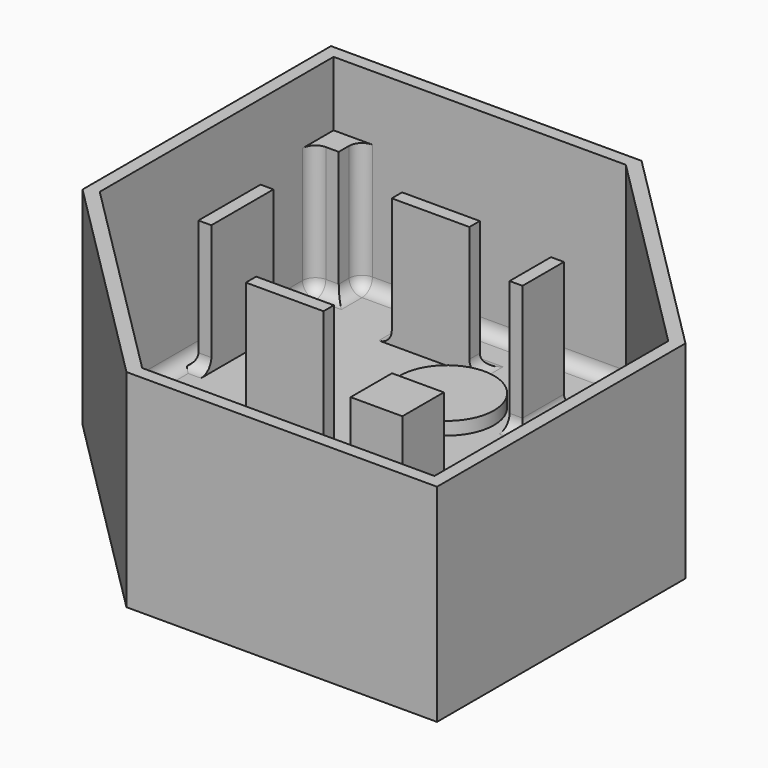
from build123d import *

# Parameters (mm, degrees)
F1_DEPTH      = 50.8
F2_T          = -3.175
F3_W          = 19.05
F3_H          = 3.175
F3_W_2        = 3.175
F3_H_2        = 19.05
F3_H_3        = 12.7
F3_W_3        = 12.7
F3_W_4        = 6.35
F3_H_4        = 6.35
F4_DEPTH      = 31.75
F5_R          = 11.557
F6_DEPTH      = 3.175
F7_T1_DEPTH   = 12.7
F7_T3_DEPTH   = 3.175
F7_T5_DEPTH   = 19.05
F7_T7_DEPTH   = 3.175
F7_T9_DEPTH   = 3.175
F7_T11_DEPTH  = 19.05
F7_T13_DEPTH  = 3.175
F7_T15_DEPTH  = 12.7
F7_T17_DEPTH  = 12.7
F7_T19_DEPTH  = 3.175
F7_T21_DEPTH  = 3.175
F7_T23_DEPTH  = 3.175
F7_T25_DEPTH  = 3.175
F7_T27_DEPTH  = 28.575
F7_S31_W      = 3.2385
F7_S31_H      = 3.2385
F7_T32_DEPTH  = 3.2385
F7_S37_W      = 3.2385
F7_S37_H      = 3.2385
F7_T38_DEPTH  = 3.2385
F7_S43_W      = 3.2385
F7_S43_H      = 3.2385
F7_T44_DEPTH  = 3.2385
F7_S49_W      = 3.2385
F7_S49_H      = 3.2385
F7_T50_DEPTH  = 3.2385
F7_T56_DEPTH  = 70.1223719395
F7_T61_DEPTH  = 89.4447438789
F7_T67_DEPTH  = 70.1223719395
F7_T72_DEPTH  = 70.1223719395
F7_T77_DEPTH  = 89.4447438789
F7_T83_DEPTH  = 70.1223719395
F7_T89_DEPTH  = 11.1125
F7_T93_DEPTH  = 20.6375
F7_T100_DEPTH = 11.1125
F7_T104_DEPTH = 20.6375
F7_T111_DEPTH = 26.9875
F7_T115_DEPTH = 11.1125
F7_T122_DEPTH = 26.9875
F7_T126_DEPTH = 11.1125
F7_T133_DEPTH = 26.9875
F7_T137_DEPTH = 11.1125
F7_T145_DEPTH = 26.9875
F7_T149_DEPTH = 11.1125
F7_T157_DEPTH = 11.1125
F7_T161_DEPTH = 26.9875
F7_T168_DEPTH = 26.9875
F7_T172_DEPTH = 11.1125
F7_T179_DEPTH = 20.6375
F7_T183_DEPTH = 20.6375
F7_T190_DEPTH = 20.6375
F7_T194_DEPTH = 20.6375
F7_T201_DEPTH = 20.6375
F7_T205_DEPTH = 20.6375
F7_T212_DEPTH = 20.6375
F7_T216_DEPTH = 20.6375
F7_T223_DEPTH = 11.1125
F7_T227_DEPTH = 11.1125
F7_T234_DEPTH = 11.1125
F7_T238_DEPTH = 11.1125


# Not quite as in the source:
# - a fillet or chamfer that OpenCascade refuses, or shapes differently, is made with other operations: its cross-section is extruded or revolved along the edge and cut away or added


with BuildPart() as f1:
    # F0 (on Top) → F1 (new body)
    with BuildSketch(Plane.XY):
        Polygon((-53.8815367264, 53.8815367264), (0, 0), (76.2, 0), (76.2, 76.2), (22.3184632736, 130.0815367264), (-53.8815367264, 130.0815367264), align=None)
    extrude(amount=F1_DEPTH)

    # F2
    f2_openings = [f1.faces().sort_by_distance(p)[0] for p in [
        (11.159232, 65.040768, 50.8),
    ]]
    offset(amount=F2_T, openings=f2_openings)

    # F3 (on face) → F4 (join)
    with BuildSketch(Plane.XY.offset(3.175)):
        with Locations((-14.8516007567, 113.4290007567)):
            Rectangle(F3_W, F3_H)
        with Locations((-14.8516007567, 68.6742007567)):
            Rectangle(F3_W, F3_H)
        with Locations((-45.9793007567, 91.0516007567)):
            Rectangle(F3_W_2, F3_H_2)
        with Locations((16.2760992433, 105.4915007567)):
            Rectangle(F3_W_2, F3_H_3)
        with Locations((27.3533352131, 48.8466647869)):
            Rectangle(F3_W_3, F3_H_3)
        with Locations((69.85, 6.35)):
            Rectangle(F3_W_4, F3_H_4)
        with Locations((-47.5315367264, 123.7315367264)):
            Rectangle(F3_W_4, F3_H_4)
    extrude(amount=F4_DEPTH)

    # F5 (on face) → F6 (join)
    with BuildSketch(Plane.XY.offset(3.175)):
        with Locations((0.0581992433, 98.2017007567)):
            Circle(F5_R)
    extrude(amount=F6_DEPTH)

    # F7: fillet of radius 3.175 on 30 edges, made by hand

    # F7_s2 → F7_t1 (join)
    with BuildSketch(Plane.XZ.offset(-111.8415007567)):
        with BuildLine():
            ThreePointArc((21.0385992433, 3.175), (18.7935352131, 4.1049359697), (17.8635992433, 6.35))
            Line((17.8635992433, 6.35), (17.8635992433, 3.175))
            Line((17.8635992433, 3.175), (21.0385992433, 3.175))
        make_face()
    extrude(amount=F7_T1_DEPTH)

    # F7_s4 → F7_t3 (join)
    with BuildSketch(Plane.YZ.offset(14.6885992433)):
        with BuildLine():
            ThreePointArc((115.0165007567, 3.175), (112.7714367264, 4.1049359697), (111.8415007567, 6.35))
            Line((111.8415007567, 6.35), (111.8415007567, 3.175))
            Line((111.8415007567, 3.175), (115.0165007567, 3.175))
        make_face()
        with BuildLine():
            ThreePointArc((95.9665007567, 3.175), (98.2115647869, 4.1049359697), (99.1415007567, 6.35))
            Line((99.1415007567, 6.35), (99.1415007567, 3.175))
            Line((99.1415007567, 3.175), (95.9665007567, 3.175))
        make_face()
    extrude(amount=F7_T3_DEPTH)

    # F7_s6 → F7_t5 (join)
    with BuildSketch(Plane.YZ.offset(-24.3766007567)):
        with BuildLine():
            ThreePointArc((63.9117007567, 3.175), (66.1567647869, 4.1049359697), (67.0867007567, 6.35))
            Line((67.0867007567, 6.35), (67.0867007567, 3.175))
            Line((67.0867007567, 3.175), (63.9117007567, 3.175))
        make_face()
        with BuildLine():
            ThreePointArc((118.1915007567, 3.175), (115.9464367264, 4.1049359697), (115.0165007567, 6.35))
            Line((115.0165007567, 6.35), (115.0165007567, 3.175))
            Line((115.0165007567, 3.175), (118.1915007567, 3.175))
        make_face()
    extrude(amount=F7_T5_DEPTH)

    # F7_s8 → F7_t7 (join)
    with BuildSketch(Plane.XZ.offset(-70.2617007567)):
        with BuildLine():
            ThreePointArc((-2.1516007567, 3.175), (-4.3966647869, 4.1049359697), (-5.3266007567, 6.35))
            Line((-5.3266007567, 6.35), (-5.3266007567, 3.175))
            Line((-5.3266007567, 3.175), (-2.1516007567, 3.175))
        make_face()
        with BuildLine():
            ThreePointArc((-27.5516007567, 3.175), (-25.3065367264, 4.1049359697), (-24.3766007567, 6.35))
            Line((-24.3766007567, 6.35), (-24.3766007567, 3.175))
            Line((-24.3766007567, 3.175), (-27.5516007567, 3.175))
        make_face()
    extrude(amount=F7_T7_DEPTH)

    # F7_s10 → F7_t9 (join)
    with BuildSketch(Plane.YZ.offset(-47.5668007567)):
        with BuildLine():
            ThreePointArc((78.3516007567, 3.175), (80.5966647869, 4.1049359697), (81.5266007567, 6.35))
            Line((81.5266007567, 6.35), (81.5266007567, 3.175))
            Line((81.5266007567, 3.175), (78.3516007567, 3.175))
        make_face()
        with BuildLine():
            ThreePointArc((103.7516007567, 3.175), (101.5065367264, 4.1049359697), (100.5766007567, 6.35))
            Line((100.5766007567, 6.35), (100.5766007567, 3.175))
            Line((100.5766007567, 3.175), (103.7516007567, 3.175))
        make_face()
    extrude(amount=F7_T9_DEPTH)

    # F7_s12 → F7_t11 (join)
    with BuildSketch(Plane.XZ.offset(-100.5766007567)):
        with BuildLine():
            ThreePointArc((-50.7418007567, 3.175), (-48.4967367264, 4.1049359697), (-47.5668007567, 6.35))
            Line((-47.5668007567, 6.35), (-47.5668007567, 3.175))
            Line((-47.5668007567, 3.175), (-50.7418007567, 3.175))
        make_face()
    extrude(amount=F7_T11_DEPTH)

    # F7_s14 → F7_t13 (join)
    with BuildSketch(Plane.XZ.offset(-115.0165007567)):
        with BuildLine():
            ThreePointArc((-27.5516007567, 3.175), (-25.3065367264, 4.1049359697), (-24.3766007567, 6.35))
            Line((-24.3766007567, 6.35), (-24.3766007567, 3.175))
            Line((-24.3766007567, 3.175), (-27.5516007567, 3.175))
        make_face()
        with BuildLine():
            ThreePointArc((-2.1516007567, 3.175), (-4.3966647869, 4.1049359697), (-5.3266007567, 6.35))
            Line((-5.3266007567, 6.35), (-5.3266007567, 3.175))
            Line((-5.3266007567, 3.175), (-2.1516007567, 3.175))
        make_face()
    extrude(amount=F7_T13_DEPTH)

    # F7_s16 → F7_t15 (join)
    with BuildSketch(Plane.YZ.offset(21.0033352131)):
        with BuildLine():
            ThreePointArc((58.3716647869, 3.175), (56.1266007567, 4.1049359697), (55.1966647869, 6.35))
            Line((55.1966647869, 6.35), (55.1966647869, 3.175))
            Line((55.1966647869, 3.175), (58.3716647869, 3.175))
        make_face()
        with BuildLine():
            ThreePointArc((39.3216647869, 3.175), (41.5667288172, 4.1049359697), (42.4966647869, 6.35))
            Line((42.4966647869, 6.35), (42.4966647869, 3.175))
            Line((42.4966647869, 3.175), (39.3216647869, 3.175))
        make_face()
    extrude(amount=F7_T15_DEPTH)

    # F7_s18 → F7_t17 (join)
    with BuildSketch(Plane.XZ.offset(-55.1966647869)):
        with BuildLine():
            ThreePointArc((36.8783352131, 3.175), (34.6332711828, 4.1049359697), (33.7033352131, 6.35))
            Line((33.7033352131, 6.35), (33.7033352131, 3.175))
            Line((33.7033352131, 3.175), (36.8783352131, 3.175))
        make_face()
        with BuildLine():
            ThreePointArc((17.8283352131, 3.175), (20.0733992433, 4.1049359697), (21.0033352131, 6.35))
            Line((21.0033352131, 6.35), (21.0033352131, 3.175))
            Line((21.0033352131, 3.175), (17.8283352131, 3.175))
        make_face()
    extrude(amount=F7_T17_DEPTH)

    # F7_s20 → F7_t19 (join)
    with BuildSketch(Plane.YZ.offset(-47.5315367264)):
        with BuildLine():
            ThreePointArc((117.3815367264, 3.175), (119.6266007567, 4.1049359697), (120.5565367264, 6.35))
            Line((120.5565367264, 6.35), (120.5565367264, 3.175))
            Line((120.5565367264, 3.175), (117.3815367264, 3.175))
        make_face()
    extrude(amount=F7_T19_DEPTH)

    # F7_s22 → F7_t21 (join)
    with BuildSketch(Plane.XZ.offset(-123.7315367264)):
        with BuildLine():
            ThreePointArc((-41.1815367264, 3.175), (-43.4266007567, 4.1049359697), (-44.3565367264, 6.35))
            Line((-44.3565367264, 6.35), (-44.3565367264, 3.175))
            Line((-44.3565367264, 3.175), (-41.1815367264, 3.175))
        make_face()
    extrude(amount=F7_T21_DEPTH)

    # F7_s24 → F7_t23 (join)
    with BuildSketch(Plane.YZ.offset(66.675)):
        with BuildLine():
            ThreePointArc((12.7, 3.175), (10.4549359697, 4.1049359697), (9.525, 6.35))
            Line((9.525, 6.35), (9.525, 3.175))
            Line((9.525, 3.175), (12.7, 3.175))
        make_face()
    extrude(amount=F7_T23_DEPTH)

    # F7_s26 → F7_t25 (join)
    with BuildSketch(Plane.XZ.offset(-9.525)):
        with BuildLine():
            ThreePointArc((63.5, 3.175), (65.7450640303, 4.1049359697), (66.675, 6.35))
            Line((66.675, 6.35), (66.675, 3.175))
            Line((66.675, 3.175), (63.5, 3.175))
        make_face()
    extrude(amount=F7_T25_DEPTH)

    # F7_s28 → F7_t27 (join)
    with BuildSketch(Plane.XY.offset(6.35)):
        with BuildLine():
            ThreePointArc((-50.7065367264, 117.3815367264), (-49.7766007567, 119.6266007567), (-47.5315367264, 120.5565367264))
            Line((-47.5315367264, 120.5565367264), (-50.7065367264, 120.5565367264))
            Line((-50.7065367264, 120.5565367264), (-50.7065367264, 117.3815367264))
        make_face()
        with BuildLine():
            ThreePointArc((-41.1815367264, 126.9065367264), (-43.4266007567, 125.9766007567), (-44.3565367264, 123.7315367264))
            Line((-44.3565367264, 123.7315367264), (-44.3565367264, 126.9065367264))
            Line((-44.3565367264, 126.9065367264), (-41.1815367264, 126.9065367264))
        make_face()
        with BuildLine():
            ThreePointArc((73.025, 12.7), (72.0950640303, 10.4549359697), (69.85, 9.525))
            Line((69.85, 9.525), (73.025, 9.525))
            Line((73.025, 9.525), (73.025, 12.7))
        make_face()
        with BuildLine():
            ThreePointArc((63.5, 3.175), (65.7450640303, 4.1049359697), (66.675, 6.35))
            Line((66.675, 6.35), (66.675, 3.175))
            Line((66.675, 3.175), (63.5, 3.175))
        make_face()
    extrude(amount=F7_T27_DEPTH)


with BuildPart() as f7_tool30:
    # F7_s31 → F7_t32 (new body)
    with BuildSketch(Plane.XZ.offset(-117.3815367264)):
        with Locations((-49.1507867264, 4.73075)):
            Rectangle(F7_S31_W, F7_S31_H)
    extrude(amount=-F7_T32_DEPTH)

    # F7_s33 → F7_t34 (revolve, cut)
    with BuildSketch(Plane(origin=(-47.5315367264, 117.3815367264, 6.35), x_dir=(0.7071067812, 0, 0.7071067812), z_dir=(-0.7071067812, 0, 0.7071067812))):
        with BuildLine():
            ThreePointArc((0, -3.175), (3.175, 0), (0, 3.175))
            Line((0, 3.175), (0, -3.175))
        make_face()
    revolve(axis=Axis((-47.5315367264, 117.3815367264, 6.35), (0, 1, 0)), mode=Mode.SUBTRACT)


with BuildPart() as f1_1:
    add(f1.part)

    # F7_t29: union F7_tool30
    add(f7_tool30.part)


with BuildPart() as f7_tool36:
    # F7_s37 → F7_t38 (new body)
    with BuildSketch(Plane.YZ.offset(-41.1815367264)):
        with Locations((125.3507867264, 4.73075)):
            Rectangle(F7_S37_W, F7_S37_H)
    extrude(amount=-F7_T38_DEPTH)

    # F7_s39 → F7_t40 (revolve, cut)
    with BuildSketch(Plane(origin=(-41.1815367264, 123.7315367264, 6.35), x_dir=(0, -0.7071067812, 0.7071067812), z_dir=(0, -0.7071067812, -0.7071067812))):
        with BuildLine():
            ThreePointArc((0, -3.175), (3.175, 0), (0, 3.175))
            Line((0, 3.175), (0, -3.175))
        make_face()
    revolve(axis=Axis((-41.1815367264, 123.7315367264, 6.35), (-1, 0, 0)), mode=Mode.SUBTRACT)


with BuildPart() as f1_2:
    add(f1_1.part)

    # F7_t35: union F7_tool36
    add(f7_tool36.part)


with BuildPart() as f7_tool42:
    # F7_s43 → F7_t44 (new body)
    with BuildSketch(Plane.XZ.offset(-12.7)):
        with Locations((71.46925, 4.73075)):
            Rectangle(F7_S43_W, F7_S43_H)
    extrude(amount=F7_T44_DEPTH)

    # F7_s45 → F7_t46 (revolve, cut)
    with BuildSketch(Plane(origin=(69.85, 12.7, 6.35), x_dir=(-0.7071067812, 0, 0.7071067812), z_dir=(0.7071067812, 0, 0.7071067812))):
        with BuildLine():
            ThreePointArc((0, -3.175), (3.175, 0), (0, 3.175))
            Line((0, 3.175), (0, -3.175))
        make_face()
    revolve(axis=Axis((69.85, 12.7, 6.35), (0, -1, 0)), mode=Mode.SUBTRACT)


with BuildPart() as f1_3:
    add(f1_2.part)

    # F7_t41: union F7_tool42
    add(f7_tool42.part)


with BuildPart() as f7_tool48:
    # F7_s49 → F7_t50 (new body)
    with BuildSketch(Plane.YZ.offset(63.5)):
        with Locations((4.73075, 4.73075)):
            Rectangle(F7_S49_W, F7_S49_H)
    extrude(amount=F7_T50_DEPTH)

    # F7_s51 → F7_t52 (revolve, cut)
    with BuildSketch(Plane(origin=(63.5, 6.35, 6.35), x_dir=(0, 0.7071067812, 0.7071067812), z_dir=(0, 0.7071067812, -0.7071067812))):
        with BuildLine():
            ThreePointArc((0, -3.175), (3.175, 0), (0, 3.175))
            Line((0, 3.175), (0, -3.175))
        make_face()
    revolve(axis=Axis((63.5, 6.35, 6.35), (1, 0, 0)), mode=Mode.SUBTRACT)


with BuildPart() as f1_4:
    add(f1_3.part)

    # F7_t47: union F7_tool48
    add(f7_tool48.part)


with BuildPart() as f7_tool54:
    # F7_s55 → F7_t56 (new body)
    with BuildSketch(Plane.YZ.offset(28.9408352131)):
        with BuildLine():
            ThreePointArc((126.9065367264, 6.35), (125.9766007567, 4.1049359697), (123.7315367264, 3.175))
            Line((123.7315367264, 3.175), (126.9065367264, 3.175))
            Line((126.9065367264, 3.175), (126.9065367264, 6.35))
        make_face()
    extrude(amount=-F7_T56_DEPTH)

    split(bisect_by=Plane(origin=(73.9549359697, 73.9549359697, 0), x_dir=(0, 0, 1), z_dir=(-0.7071067812, -0.7071067812, 0)), keep=Keep.TOP)


with BuildPart() as f1_5:
    add(f1_4.part)

    # F7_t53: union F7_tool54
    add(f7_tool54.part)


with BuildPart() as f7_tool59:
    # F7_s60 → F7_t61 (new body)
    with BuildSketch(Plane(origin=(4.6827241059, -4.6827241059, 0), x_dir=(0, 0, 1), z_dir=(-0.7071067812, 0.7071067812, 0))):
        with BuildLine():
            ThreePointArc((6.35, 104.5880734528), (4.1049359697, 103.6581374831), (3.175, 101.4130734528))
            Line((3.175, 101.4130734528), (3.175, 104.5880734528))
            Line((3.175, 104.5880734528), (6.35, 104.5880734528))
        make_face()
    extrude(amount=F7_T61_DEPTH)

    split(bisect_by=Plane.XZ.offset(-126.9065367264), keep=Keep.TOP)

    split(bisect_by=Plane.YZ.offset(73.025), keep=Keep.BOTTOM)


with BuildPart() as f1_6:
    add(f1_5.part)

    # F7_t58: union F7_tool59
    add(f7_tool59.part)


with BuildPart() as f7_tool65:
    # F7_s66 → F7_t67 (new body)
    with BuildSketch(Plane.XZ.offset(-12.7)):
        with BuildLine():
            ThreePointArc((73.025, 6.35), (72.0950640303, 4.1049359697), (69.85, 3.175))
            Line((69.85, 3.175), (73.025, 3.175))
            Line((73.025, 3.175), (73.025, 6.35))
        make_face()
    extrude(amount=-F7_T67_DEPTH)

    split(bisect_by=Plane(origin=(73.9549359697, 73.9549359697, 0), x_dir=(0, 0, 1), z_dir=(-0.7071067812, -0.7071067812, 0)), keep=Keep.TOP)


with BuildPart() as f1_7:
    add(f1_6.part)

    # F7_t64: union F7_tool65
    add(f7_tool65.part)


with BuildPart() as f7_tool70:
    # F7_s71 → F7_t72 (new body)
    with BuildSketch(Plane.YZ.offset(-6.6223719395)):
        with BuildLine():
            ThreePointArc((3.175, 6.35), (4.1049359697, 4.1049359697), (6.35, 3.175))
            Line((6.35, 3.175), (3.175, 3.175))
            Line((3.175, 3.175), (3.175, 6.35))
        make_face()
    extrude(amount=F7_T72_DEPTH)

    split(bisect_by=Plane(origin=(2.2450640303, 2.2450640303, 0), x_dir=(0, 0, 1), z_dir=(0.7071067812, 0.7071067812, 0)), keep=Keep.TOP)


with BuildPart() as f1_8:
    add(f1_7.part)

    # F7_t69: union F7_tool70
    add(f7_tool70.part)


with BuildPart() as f7_tool75:
    # F7_s76 → F7_t77 (new body)
    with BuildSketch(Plane(origin=(-58.5642608324, 58.5642608324, 0), x_dir=(0, 0, 1), z_dir=(0.7071067812, -0.7071067812, 0))):
        with BuildLine():
            ThreePointArc((6.35, -3.175), (4.1049359697, -4.1049359697), (3.175, -6.35))
            Line((3.175, -6.35), (3.175, -3.175))
            Line((3.175, -3.175), (6.35, -3.175))
        make_face()
    extrude(amount=F7_T77_DEPTH)

    split(bisect_by=Plane.YZ.offset(-50.7065367264), keep=Keep.TOP)

    split(bisect_by=Plane.XZ.offset(-3.175), keep=Keep.BOTTOM)


with BuildPart() as f1_9:
    add(f1_8.part)

    # F7_t74: union F7_tool75
    add(f7_tool75.part)


with BuildPart() as f7_tool81:
    # F7_s82 → F7_t83 (new body)
    with BuildSketch(Plane.XZ.offset(-117.3815367264)):
        with BuildLine():
            ThreePointArc((-50.7065367264, 6.35), (-49.7766007567, 4.1049359697), (-47.5315367264, 3.175))
            Line((-47.5315367264, 3.175), (-50.7065367264, 3.175))
            Line((-50.7065367264, 3.175), (-50.7065367264, 6.35))
        make_face()
    extrude(amount=F7_T83_DEPTH)

    split(bisect_by=Plane(origin=(2.2450640303, 2.2450640303, 0), x_dir=(0, 0, 1), z_dir=(0.7071067812, 0.7071067812, 0)), keep=Keep.TOP)


with BuildPart() as f1_10:
    add(f1_9.part)

    # F7_t80: union F7_tool81
    add(f7_tool81.part)


with BuildPart() as f7_tool87:
    # F7_s88 → F7_t89 (new body)
    with BuildSketch(Plane.YZ.offset(14.6885992433)):
        with BuildLine():
            ThreePointArc((95.9665007567, 3.175), (98.2115647869, 4.1049359697), (99.1415007567, 6.35))
            Line((99.1415007567, 6.35), (99.1415007567, 3.175))
            Line((99.1415007567, 3.175), (95.9665007567, 3.175))
        make_face()
    extrude(amount=F7_T89_DEPTH)

    split(bisect_by=Plane.YZ.offset(17.8635992433), keep=Keep.TOP)


with BuildPart() as f7_tool91:
    # F7_s92 → F7_t93 (new body)
    with BuildSketch(Plane.XZ.offset(-91.2040007567)):
        with BuildLine():
            ThreePointArc((21.0385992433, 3.175), (18.7935352131, 4.1049359697), (17.8635992433, 6.35))
            Line((17.8635992433, 6.35), (17.8635992433, 3.175))
            Line((17.8635992433, 3.175), (21.0385992433, 3.175))
        make_face()
    extrude(amount=-F7_T93_DEPTH)

    split(bisect_by=Plane.XZ.offset(-99.1415007567), keep=Keep.TOP)


with BuildPart() as f7_tool87_1:
    add(f7_tool87.part)

    # F7_t95: intersect F7_tool91
    add(f7_tool91.part, mode=Mode.INTERSECT)


with BuildPart() as f1_11:
    add(f1_10.part)

    # F7_t85: union F7_tool87
    add(f7_tool87_1.part)


with BuildPart() as f7_tool98:
    # F7_s99 → F7_t100 (new body)
    with BuildSketch(Plane.YZ.offset(25.8010992433)):
        with BuildLine():
            ThreePointArc((115.0165007567, 3.175), (112.7714367264, 4.1049359697), (111.8415007567, 6.35))
            Line((111.8415007567, 6.35), (111.8415007567, 3.175))
            Line((111.8415007567, 3.175), (115.0165007567, 3.175))
        make_face()
    extrude(amount=-F7_T100_DEPTH)

    split(bisect_by=Plane.YZ.offset(17.8635992433), keep=Keep.TOP)


with BuildPart() as f7_tool102:
    # F7_s103 → F7_t104 (new body)
    with BuildSketch(Plane.XZ.offset(-99.1415007567)):
        with BuildLine():
            ThreePointArc((21.0385992433, 3.175), (18.7935352131, 4.1049359697), (17.8635992433, 6.35))
            Line((17.8635992433, 6.35), (17.8635992433, 3.175))
            Line((17.8635992433, 3.175), (21.0385992433, 3.175))
        make_face()
    extrude(amount=-F7_T104_DEPTH)

    split(bisect_by=Plane.XZ.offset(-111.8415007567), keep=Keep.BOTTOM)


with BuildPart() as f7_tool98_1:
    add(f7_tool98.part)

    # F7_t106: intersect F7_tool102
    add(f7_tool102.part, mode=Mode.INTERSECT)


with BuildPart() as f1_12:
    add(f1_11.part)

    # F7_t96: union F7_tool98
    add(f7_tool98_1.part)


with BuildPart() as f7_tool109:
    # F7_s110 → F7_t111 (new body)
    with BuildSketch(Plane.YZ.offset(-32.3141007567)):
        with BuildLine():
            ThreePointArc((63.9117007567, 3.175), (66.1567647869, 4.1049359697), (67.0867007567, 6.35))
            Line((67.0867007567, 6.35), (67.0867007567, 3.175))
            Line((67.0867007567, 3.175), (63.9117007567, 3.175))
        make_face()
    extrude(amount=F7_T111_DEPTH)

    split(bisect_by=Plane.YZ.offset(-24.3766007567), keep=Keep.BOTTOM)


with BuildPart() as f7_tool113:
    # F7_s114 → F7_t115 (new body)
    with BuildSketch(Plane.XZ.offset(-70.2617007567)):
        with BuildLine():
            ThreePointArc((-27.5516007567, 3.175), (-25.3065367264, 4.1049359697), (-24.3766007567, 6.35))
            Line((-24.3766007567, 6.35), (-24.3766007567, 3.175))
            Line((-24.3766007567, 3.175), (-27.5516007567, 3.175))
        make_face()
    extrude(amount=F7_T115_DEPTH)

    split(bisect_by=Plane.XZ.offset(-67.0867007567), keep=Keep.TOP)


with BuildPart() as f7_tool109_1:
    add(f7_tool109.part)

    # F7_t117: intersect F7_tool113
    add(f7_tool113.part, mode=Mode.INTERSECT)


with BuildPart() as f1_13:
    add(f1_12.part)

    # F7_t107: union F7_tool109
    add(f7_tool109_1.part)


with BuildPart() as f7_tool120:
    # F7_s121 → F7_t122 (new body)
    with BuildSketch(Plane.YZ.offset(-24.3766007567)):
        with BuildLine():
            ThreePointArc((63.9117007567, 3.175), (66.1567647869, 4.1049359697), (67.0867007567, 6.35))
            Line((67.0867007567, 6.35), (67.0867007567, 3.175))
            Line((67.0867007567, 3.175), (63.9117007567, 3.175))
        make_face()
    extrude(amount=F7_T122_DEPTH)

    split(bisect_by=Plane.YZ.offset(-5.3266007567), keep=Keep.TOP)


with BuildPart() as f7_tool124:
    # F7_s125 → F7_t126 (new body)
    with BuildSketch(Plane.XZ.offset(-59.1492007567)):
        with BuildLine():
            ThreePointArc((-2.1516007567, 3.175), (-4.3966647869, 4.1049359697), (-5.3266007567, 6.35))
            Line((-5.3266007567, 6.35), (-5.3266007567, 3.175))
            Line((-5.3266007567, 3.175), (-2.1516007567, 3.175))
        make_face()
    extrude(amount=-F7_T126_DEPTH)

    split(bisect_by=Plane.XZ.offset(-67.0867007567), keep=Keep.TOP)


with BuildPart() as f7_tool120_1:
    add(f7_tool120.part)

    # F7_t128: intersect F7_tool124
    add(f7_tool124.part, mode=Mode.INTERSECT)


with BuildPart() as f1_14:
    add(f1_13.part)

    # F7_t118: union F7_tool120
    add(f7_tool120_1.part)


with BuildPart() as f7_tool131:
    # F7_s132 → F7_t133 (new body)
    with BuildSketch(Plane.XZ.offset(-100.5766007567)):
        with BuildLine():
            ThreePointArc((-50.7418007567, 3.175), (-48.4967367264, 4.1049359697), (-47.5668007567, 6.35))
            Line((-47.5668007567, 6.35), (-47.5668007567, 3.175))
            Line((-47.5668007567, 3.175), (-50.7418007567, 3.175))
        make_face()
    extrude(amount=F7_T133_DEPTH)

    split(bisect_by=Plane.XZ.offset(-81.5266007567), keep=Keep.TOP)


with BuildPart() as f7_tool135:
    # F7_s136 → F7_t137 (new body)
    with BuildSketch(Plane.YZ.offset(-55.5043007567)):
        with BuildLine():
            ThreePointArc((78.3516007567, 3.175), (80.5966647869, 4.1049359697), (81.5266007567, 6.35))
            Line((81.5266007567, 6.35), (81.5266007567, 3.175))
            Line((81.5266007567, 3.175), (78.3516007567, 3.175))
        make_face()
    extrude(amount=F7_T137_DEPTH)

    split(bisect_by=Plane.YZ.offset(-50.7065367264), keep=Keep.TOP)

    split(bisect_by=Plane.YZ.offset(-47.5668007567), keep=Keep.BOTTOM)


with BuildPart() as f7_tool131_1:
    add(f7_tool131.part)

    # F7_t140: intersect F7_tool135
    add(f7_tool135.part, mode=Mode.INTERSECT)


with BuildPart() as f1_15:
    add(f1_14.part)

    # F7_t129: union F7_tool131
    add(f7_tool131_1.part)


with BuildPart() as f7_tool143:
    # F7_s144 → F7_t145 (new body)
    with BuildSketch(Plane.XZ.offset(-108.5141007567)):
        with BuildLine():
            ThreePointArc((-50.7418007567, 3.175), (-48.4967367264, 4.1049359697), (-47.5668007567, 6.35))
            Line((-47.5668007567, 6.35), (-47.5668007567, 3.175))
            Line((-47.5668007567, 3.175), (-50.7418007567, 3.175))
        make_face()
    extrude(amount=F7_T145_DEPTH)

    split(bisect_by=Plane.XZ.offset(-100.5766007567), keep=Keep.BOTTOM)


with BuildPart() as f7_tool147:
    # F7_s148 → F7_t149 (new body)
    with BuildSketch(Plane.YZ.offset(-44.3918007567)):
        with BuildLine():
            ThreePointArc((103.7516007567, 3.175), (101.5065367264, 4.1049359697), (100.5766007567, 6.35))
            Line((100.5766007567, 6.35), (100.5766007567, 3.175))
            Line((100.5766007567, 3.175), (103.7516007567, 3.175))
        make_face()
    extrude(amount=-F7_T149_DEPTH)

    split(bisect_by=Plane.YZ.offset(-50.7065367264), keep=Keep.TOP)

    split(bisect_by=Plane.YZ.offset(-47.5668007567), keep=Keep.BOTTOM)


with BuildPart() as f7_tool143_1:
    add(f7_tool143.part)

    # F7_t152: intersect F7_tool147
    add(f7_tool147.part, mode=Mode.INTERSECT)


with BuildPart() as f1_16:
    add(f1_15.part)

    # F7_t141: union F7_tool143
    add(f7_tool143_1.part)


with BuildPart() as f7_tool155:
    # F7_s156 → F7_t157 (new body)
    with BuildSketch(Plane.XZ.offset(-122.9540007567)):
        with BuildLine():
            ThreePointArc((-27.5516007567, 3.175), (-25.3065367264, 4.1049359697), (-24.3766007567, 6.35))
            Line((-24.3766007567, 6.35), (-24.3766007567, 3.175))
            Line((-24.3766007567, 3.175), (-27.5516007567, 3.175))
        make_face()
    extrude(amount=F7_T157_DEPTH)

    split(bisect_by=Plane.XZ.offset(-115.0165007567), keep=Keep.BOTTOM)


with BuildPart() as f7_tool159:
    # F7_s160 → F7_t161 (new body)
    with BuildSketch(Plane.YZ.offset(-5.3266007567)):
        with BuildLine():
            ThreePointArc((118.1915007567, 3.175), (115.9464367264, 4.1049359697), (115.0165007567, 6.35))
            Line((115.0165007567, 6.35), (115.0165007567, 3.175))
            Line((115.0165007567, 3.175), (118.1915007567, 3.175))
        make_face()
    extrude(amount=-F7_T161_DEPTH)

    split(bisect_by=Plane.YZ.offset(-24.3766007567), keep=Keep.BOTTOM)


with BuildPart() as f7_tool155_1:
    add(f7_tool155.part)

    # F7_t163: intersect F7_tool159
    add(f7_tool159.part, mode=Mode.INTERSECT)


with BuildPart() as f1_17:
    add(f1_16.part)

    # F7_t153: union F7_tool155
    add(f7_tool155_1.part)


with BuildPart() as f7_tool166:
    # F7_s167 → F7_t168 (new body)
    with BuildSketch(Plane.YZ.offset(2.6108992433)):
        with BuildLine():
            ThreePointArc((118.1915007567, 3.175), (115.9464367264, 4.1049359697), (115.0165007567, 6.35))
            Line((115.0165007567, 6.35), (115.0165007567, 3.175))
            Line((115.0165007567, 3.175), (118.1915007567, 3.175))
        make_face()
    extrude(amount=-F7_T168_DEPTH)

    split(bisect_by=Plane.YZ.offset(-5.3266007567), keep=Keep.TOP)


with BuildPart() as f7_tool170:
    # F7_s171 → F7_t172 (new body)
    with BuildSketch(Plane.XZ.offset(-111.8415007567)):
        with BuildLine():
            ThreePointArc((-2.1516007567, 3.175), (-4.3966647869, 4.1049359697), (-5.3266007567, 6.35))
            Line((-5.3266007567, 6.35), (-5.3266007567, 3.175))
            Line((-5.3266007567, 3.175), (-2.1516007567, 3.175))
        make_face()
    extrude(amount=-F7_T172_DEPTH)

    split(bisect_by=Plane.XZ.offset(-115.0165007567), keep=Keep.BOTTOM)


with BuildPart() as f7_tool166_1:
    add(f7_tool166.part)

    # F7_t174: intersect F7_tool170
    add(f7_tool170.part, mode=Mode.INTERSECT)


with BuildPart() as f1_18:
    add(f1_17.part)

    # F7_t164: union F7_tool166
    add(f7_tool166_1.part)


with BuildPart() as f7_tool177:
    # F7_s178 → F7_t179 (new body)
    with BuildSketch(Plane.YZ.offset(41.6408352131)):
        with BuildLine():
            ThreePointArc((58.3716647869, 3.175), (56.1266007567, 4.1049359697), (55.1966647869, 6.35))
            Line((55.1966647869, 6.35), (55.1966647869, 3.175))
            Line((55.1966647869, 3.175), (58.3716647869, 3.175))
        make_face()
    extrude(amount=-F7_T179_DEPTH)

    split(bisect_by=Plane.YZ.offset(33.7033352131), keep=Keep.TOP)


with BuildPart() as f7_tool181:
    # F7_s182 → F7_t183 (new body)
    with BuildSketch(Plane.XZ.offset(-42.4966647869)):
        with BuildLine():
            ThreePointArc((36.8783352131, 3.175), (34.6332711828, 4.1049359697), (33.7033352131, 6.35))
            Line((33.7033352131, 6.35), (33.7033352131, 3.175))
            Line((33.7033352131, 3.175), (36.8783352131, 3.175))
        make_face()
    extrude(amount=-F7_T183_DEPTH)

    split(bisect_by=Plane.XZ.offset(-55.1966647869), keep=Keep.BOTTOM)


with BuildPart() as f7_tool177_1:
    add(f7_tool177.part)

    # F7_t185: intersect F7_tool181
    add(f7_tool181.part, mode=Mode.INTERSECT)


with BuildPart() as f1_19:
    add(f1_18.part)

    # F7_t175: union F7_tool177
    add(f7_tool177_1.part)


with BuildPart() as f7_tool188:
    # F7_s189 → F7_t190 (new body)
    with BuildSketch(Plane.YZ.offset(33.7033352131)):
        with BuildLine():
            ThreePointArc((58.3716647869, 3.175), (56.1266007567, 4.1049359697), (55.1966647869, 6.35))
            Line((55.1966647869, 6.35), (55.1966647869, 3.175))
            Line((55.1966647869, 3.175), (58.3716647869, 3.175))
        make_face()
    extrude(amount=-F7_T190_DEPTH)

    split(bisect_by=Plane.YZ.offset(21.0033352131), keep=Keep.BOTTOM)


with BuildPart() as f7_tool192:
    # F7_s193 → F7_t194 (new body)
    with BuildSketch(Plane.XZ.offset(-63.1341647869)):
        with BuildLine():
            ThreePointArc((17.8283352131, 3.175), (20.0733992433, 4.1049359697), (21.0033352131, 6.35))
            Line((21.0033352131, 6.35), (21.0033352131, 3.175))
            Line((21.0033352131, 3.175), (17.8283352131, 3.175))
        make_face()
    extrude(amount=F7_T194_DEPTH)

    split(bisect_by=Plane.XZ.offset(-55.1966647869), keep=Keep.BOTTOM)


with BuildPart() as f7_tool188_1:
    add(f7_tool188.part)

    # F7_t196: intersect F7_tool192
    add(f7_tool192.part, mode=Mode.INTERSECT)


with BuildPart() as f1_20:
    add(f1_19.part)

    # F7_t186: union F7_tool188
    add(f7_tool188_1.part)


with BuildPart() as f7_tool199:
    # F7_s200 → F7_t201 (new body)
    with BuildSketch(Plane.XZ.offset(-34.5591647869)):
        with BuildLine():
            ThreePointArc((36.8783352131, 3.175), (34.6332711828, 4.1049359697), (33.7033352131, 6.35))
            Line((33.7033352131, 6.35), (33.7033352131, 3.175))
            Line((33.7033352131, 3.175), (36.8783352131, 3.175))
        make_face()
    extrude(amount=-F7_T201_DEPTH)

    split(bisect_by=Plane.XZ.offset(-42.4966647869), keep=Keep.TOP)


with BuildPart() as f7_tool203:
    # F7_s204 → F7_t205 (new body)
    with BuildSketch(Plane.YZ.offset(21.0033352131)):
        with BuildLine():
            ThreePointArc((39.3216647869, 3.175), (41.5667288172, 4.1049359697), (42.4966647869, 6.35))
            Line((42.4966647869, 6.35), (42.4966647869, 3.175))
            Line((42.4966647869, 3.175), (39.3216647869, 3.175))
        make_face()
    extrude(amount=F7_T205_DEPTH)

    split(bisect_by=Plane.YZ.offset(33.7033352131), keep=Keep.TOP)


with BuildPart() as f7_tool199_1:
    add(f7_tool199.part)

    # F7_t207: intersect F7_tool203
    add(f7_tool203.part, mode=Mode.INTERSECT)


with BuildPart() as f1_21:
    add(f1_20.part)

    # F7_t197: union F7_tool199
    add(f7_tool199_1.part)


with BuildPart() as f7_tool210:
    # F7_s211 → F7_t212 (new body)
    with BuildSketch(Plane.XZ.offset(-55.1966647869)):
        with BuildLine():
            ThreePointArc((17.8283352131, 3.175), (20.0733992433, 4.1049359697), (21.0033352131, 6.35))
            Line((21.0033352131, 6.35), (21.0033352131, 3.175))
            Line((21.0033352131, 3.175), (17.8283352131, 3.175))
        make_face()
    extrude(amount=F7_T212_DEPTH)

    split(bisect_by=Plane.XZ.offset(-42.4966647869), keep=Keep.TOP)


with BuildPart() as f7_tool214:
    # F7_s215 → F7_t216 (new body)
    with BuildSketch(Plane.YZ.offset(13.0658352131)):
        with BuildLine():
            ThreePointArc((39.3216647869, 3.175), (41.5667288172, 4.1049359697), (42.4966647869, 6.35))
            Line((42.4966647869, 6.35), (42.4966647869, 3.175))
            Line((42.4966647869, 3.175), (39.3216647869, 3.175))
        make_face()
    extrude(amount=F7_T216_DEPTH)

    split(bisect_by=Plane.YZ.offset(21.0033352131), keep=Keep.BOTTOM)


with BuildPart() as f7_tool210_1:
    add(f7_tool210.part)

    # F7_t218: intersect F7_tool214
    add(f7_tool214.part, mode=Mode.INTERSECT)


with BuildPart() as f1_22:
    add(f1_21.part)

    # F7_t208: union F7_tool210
    add(f7_tool210_1.part)


with BuildPart() as f7_tool221:
    # F7_s222 → F7_t223 (new body)
    with BuildSketch(Plane.YZ.offset(-47.5315367264)):
        with BuildLine():
            ThreePointArc((117.3815367264, 3.175), (119.6266007567, 4.1049359697), (120.5565367264, 6.35))
            Line((120.5565367264, 6.35), (120.5565367264, 3.175))
            Line((120.5565367264, 3.175), (117.3815367264, 3.175))
        make_face()
    extrude(amount=F7_T223_DEPTH)

    split(bisect_by=Plane.YZ.offset(-44.3565367264), keep=Keep.TOP)


with BuildPart() as f7_tool225:
    # F7_s226 → F7_t227 (new body)
    with BuildSketch(Plane.XZ.offset(-112.6190367264)):
        with BuildLine():
            ThreePointArc((-41.1815367264, 3.175), (-43.4266007567, 4.1049359697), (-44.3565367264, 6.35))
            Line((-44.3565367264, 6.35), (-44.3565367264, 3.175))
            Line((-44.3565367264, 3.175), (-41.1815367264, 3.175))
        make_face()
    extrude(amount=-F7_T227_DEPTH)

    split(bisect_by=Plane.XZ.offset(-120.5565367264), keep=Keep.TOP)


with BuildPart() as f7_tool221_1:
    add(f7_tool221.part)

    # F7_t229: intersect F7_tool225
    add(f7_tool225.part, mode=Mode.INTERSECT)


with BuildPart() as f1_23:
    add(f1_22.part)

    # F7_t219: union F7_tool221
    add(f7_tool221_1.part)


with BuildPart() as f7_tool232:
    # F7_s233 → F7_t234 (new body)
    with BuildSketch(Plane.XZ.offset(-17.4625)):
        with BuildLine():
            ThreePointArc((63.5, 3.175), (65.7450640303, 4.1049359697), (66.675, 6.35))
            Line((66.675, 6.35), (66.675, 3.175))
            Line((66.675, 3.175), (63.5, 3.175))
        make_face()
    extrude(amount=F7_T234_DEPTH)

    split(bisect_by=Plane.XZ.offset(-9.525), keep=Keep.BOTTOM)


with BuildPart() as f7_tool236:
    # F7_s237 → F7_t238 (new body)
    with BuildSketch(Plane.YZ.offset(69.85)):
        with BuildLine():
            ThreePointArc((12.7, 3.175), (10.4549359697, 4.1049359697), (9.525, 6.35))
            Line((9.525, 6.35), (9.525, 3.175))
            Line((9.525, 3.175), (12.7, 3.175))
        make_face()
    extrude(amount=-F7_T238_DEPTH)

    split(bisect_by=Plane.YZ.offset(66.675), keep=Keep.BOTTOM)


with BuildPart() as f7_tool232_1:
    add(f7_tool232.part)

    # F7_t240: intersect F7_tool236
    add(f7_tool236.part, mode=Mode.INTERSECT)


with BuildPart() as f1_24:
    add(f1_23.part)

    # F7_t230: union F7_tool232
    add(f7_tool232_1.part)


solid = f1_24.part
